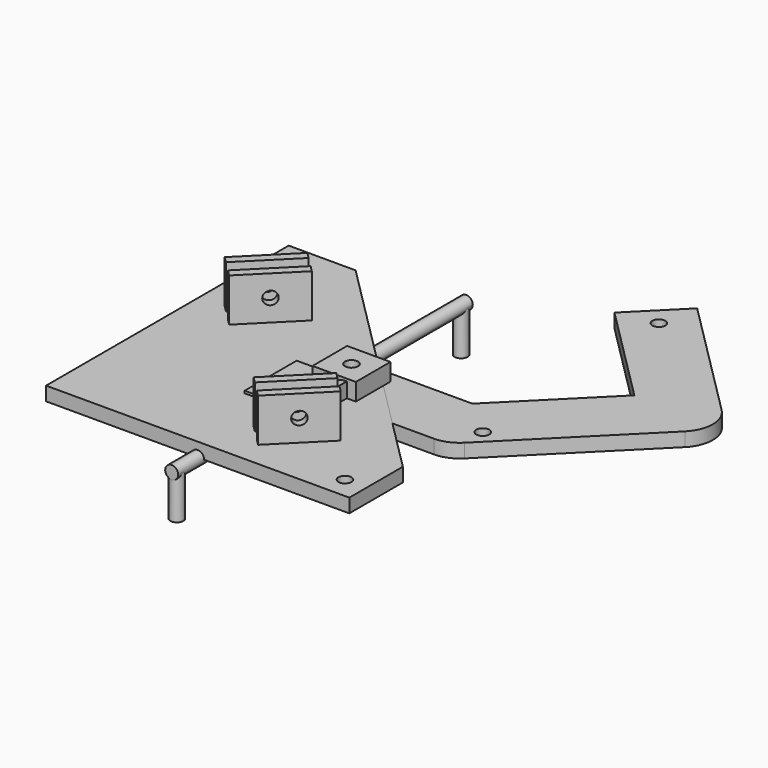
from build123d import *
from build123d import SkipClean  # not in build123d's __all__

# Parameters (mm, degrees)
F0_R      = 1.5
F1_DEPTH  = 3.2
F2_R      = 1.5
F3_DEPTH  = 3.2
F5_DEPTH  = 15
F6_R      = 1.5
F7_DEPTH  = 25
F8_R      = 5
F9_R      = 5
F10_W     = 10
F10_H     = 10
F10_R     = 1.5
F11_DEPTH = 4
F13_DEPTH = 13.2
F14_R     = 1.5
F15_DEPTH = 60
F16_R     = 1.5
F17_DEPTH = 42.5
F18_R     = 1.5
F19_DEPTH = 10
F20_R     = 1.5
F21_DEPTH = 10


with BuildPart() as f1:
    # F0 (on Top) → F1 (new body)
    with BuildSketch(Plane.XY):
        with BuildLine():
            Line((29.3933982822, 7.5), (7.5, 7.5))
            ThreePointArc((7.5, 7.5), (0, 0), (7.5, -7.5))
            Line((7.5, -7.5), (32.5, -7.5))
            ThreePointArc((32.5, -7.5), (35.3701257427, -6.9290964938), (37.8033008589, -5.3033008589))
            ThreePointArc((37.8033008589, -5.3033008589), (39.4290964938, 2.8701257427), (32.5, 7.5))
            ThreePointArc((32.5, 7.5), (29.6298742573, 6.9290964938), (27.1966991411, 5.3033008589))
            Line((27.1966991411, 5.3033008589), (29.3933982822, 7.5))
        make_face()
        with Locations((7.5, 0)):
            Circle(F0_R, mode=Mode.SUBTRACT)
        with Locations((37.8033008589, 0)):
            Circle(F0_R, mode=Mode.SUBTRACT)
        with BuildLine():
            Line((50.1776695297, 28.2842712475), (29.3933982822, 7.5))
            Line((29.3933982822, 7.5), (32.5, 7.5))
            ThreePointArc((32.5, 7.5), (39.4290964938, 2.8701257427), (37.8033008589, -5.3033008589))
            Line((37.8033008589, -5.3033008589), (66.0875721064, 22.9809703886))
            ThreePointArc((66.0875721064, 22.9809703886), (60.7842712475, 20.7842712475), (55.4809703886, 22.9809703886))
            Line((55.4809703886, 22.9809703886), (50.1776695297, 28.2842712475))
        make_face()
        with BuildLine():
            Line((32.5, 7.5), (29.3933982822, 7.5))
            Line((29.3933982822, 7.5), (27.1966991411, 5.3033008589))
            ThreePointArc((27.1966991411, 5.3033008589), (29.6298742573, 6.9290964938), (32.5, 7.5))
        make_face()
        with BuildLine():
            Line((27.1966991411, 51.265241636), (50.1776695297, 28.2842712475))
            Line((50.1776695297, 28.2842712475), (55.4809703886, 33.5875721064))
            ThreePointArc((55.4809703886, 33.5875721064), (60.7842712475, 35.7842712475), (66.0875721064, 33.5875721064))
            Line((66.0875721064, 33.5875721064), (37.8033008589, 61.8718433538))
            Line((37.8033008589, 61.8718433538), (27.1966991411, 51.265241636))
        make_face()
        with Locations((36.0355339059, 53.033008589)):
            Circle(F0_R, mode=Mode.SUBTRACT)
        with BuildLine():
            Line((55.4809703886, 33.5875721064), (50.1776695297, 28.2842712475))
            Line((50.1776695297, 28.2842712475), (55.4809703886, 22.9809703886))
            ThreePointArc((55.4809703886, 22.9809703886), (60.7842712475, 20.7842712475), (66.0875721064, 22.9809703886))
            ThreePointArc((66.0875721064, 22.9809703886), (68.2842712475, 28.2842712475), (66.0875721064, 33.5875721064))
            ThreePointArc((66.0875721064, 33.5875721064), (60.7842712475, 35.7842712475), (55.4809703886, 33.5875721064))
        make_face()
    extrude(amount=F1_DEPTH)


with BuildPart() as f3:
    # F2 (on Top) → F3 (new body)
    with BuildSketch(Plane.XY):
        Polygon((-35, -35), (35, -35), (35, -19.5508284215), (-19.5508284215, 35), (-35, 35), align=None)
        with Locations((30, -30)):
            Circle(F2_R, mode=Mode.SUBTRACT)
        with Locations((-30, 30)):
            Circle(F2_R, mode=Mode.SUBTRACT)
    extrude(amount=F3_DEPTH)

    # F12 (on face) → F13 (join)
    with BuildSketch(Plane(origin=(0, 0, 0), x_dir=(1, 0, 0), z_dir=(0, 0, -1))):
        Polygon((-17.1655729085, -18.4726088633), (-27.7721746263, -7.8660071455), (-29.1863881887, -9.2802207079), (-18.5797864709, -19.8868224257), align=None)
        Polygon((-24.0952193641, -4.1890518833), (-25.5094329265, -5.6032654457), (-14.9028312087, -16.2098671635), (-13.4886176463, -14.7956536011), align=None)
        Polygon((4.1890518833, 24.0952193641), (14.7956536011, 13.4886176463), (16.2098671635, 14.9028312087), (5.6032654457, 25.5094329265), align=None)
        Polygon((9.2802207079, 29.1863881887), (7.8660071455, 27.7721746263), (18.4726088633, 17.1655729085), (19.8868224257, 18.5797864709), align=None)
    extrude(amount=-F13_DEPTH)

    # F14 (on face) → F15 (cut)
    with BuildSketch(Plane(origin=(-19.2333044483, 19.2333044483, 0), x_dir=(-0.7071067812, -0.7071067812, 0), z_dir=(-0.7071067812, 0.7071067812, 0))):
        with Locations((6.5757860131, 8.2)):
            Circle(F14_R)
    extrude(amount=-F15_DEPTH, mode=Mode.SUBTRACT)


with BuildPart() as f5:
    # F4 (on Front) → F5 (new body)
    with BuildSketch(Plane.XZ):
        Polygon((8.4256241946, 0), (8.4256241946, -4.6235096101), (4.852652266, -1.75), (-5.147347734, -1.75), (-5.147347734, -3.75), (4.852652266, -3.75), (8.4256241946, -6.6235096101), (10.4256241946, -6.6235096101), (10.4256241946, 0), (10.4256241946, 6.6235096101), (8.4256241946, 6.6235096101), (4.852652266, 3.75), (-5.147347734, 3.75), (-5.147347734, 1.75), (4.852652266, 1.75), (8.4256241946, 4.6235096101), align=None)
    extrude(amount=F5_DEPTH)

    # F6 (on face) → F7 (cut)
    with BuildSketch(Plane.XY.offset(3.75)):
        with Locations((-2.147347734, -7.5)):
            Circle(F6_R)
    extrude(amount=-F7_DEPTH, mode=Mode.SUBTRACT)

    # F8
    f8_edges = [f5.edges().sort_by_distance(p)[0] for p in [
        (4.852652, -7.5, 3.75),
    ]]
    fillet(f8_edges, radius=F8_R)

    # F9
    f9_edges = [f5.edges().sort_by_distance(p)[0] for p in [
        (4.852652, -7.5, -3.75),
        (8.425624, -7.5, -6.62351),
        (8.425624, -7.5, 6.62351),
    ]]
    fillet(f9_edges, radius=F9_R)


with BuildPart() as f11:
    # F10 (on face) → F11 (new body)
    with BuildSketch(Plane.XY.offset(3.2)):
        with Locations((7.5, 0)):
            Rectangle(F10_W, F10_H)
        with Locations((7.5, 0)):
            Circle(F10_R, mode=Mode.SUBTRACT)
    extrude(amount=F11_DEPTH)


with BuildPart() as f17:
    # F16 (on Front) → F17 (new body, symmetric)
    with BuildSketch(Plane.XZ):
        Circle(F16_R)
    extrude(amount=F17_DEPTH, both=True)

    # F18 (on Top) → F19 (join)
    with BuildSketch(Plane.XY):
        with Locations((0, -41)):
            Circle(F18_R)
    extrude(amount=-F19_DEPTH)

    # F20 (on Top) → F21 (join)
    with BuildSketch(Plane.XY):
        with Locations((0, 41)):
            Circle(F20_R)
    with SkipClean():  # cleaning this boolean's faces spoils the solid; the shape is the same uncleaned
        extrude(amount=-F21_DEPTH)


solid = Compound([f1.part, f3.part, f5.part, f11.part, f17.part])
